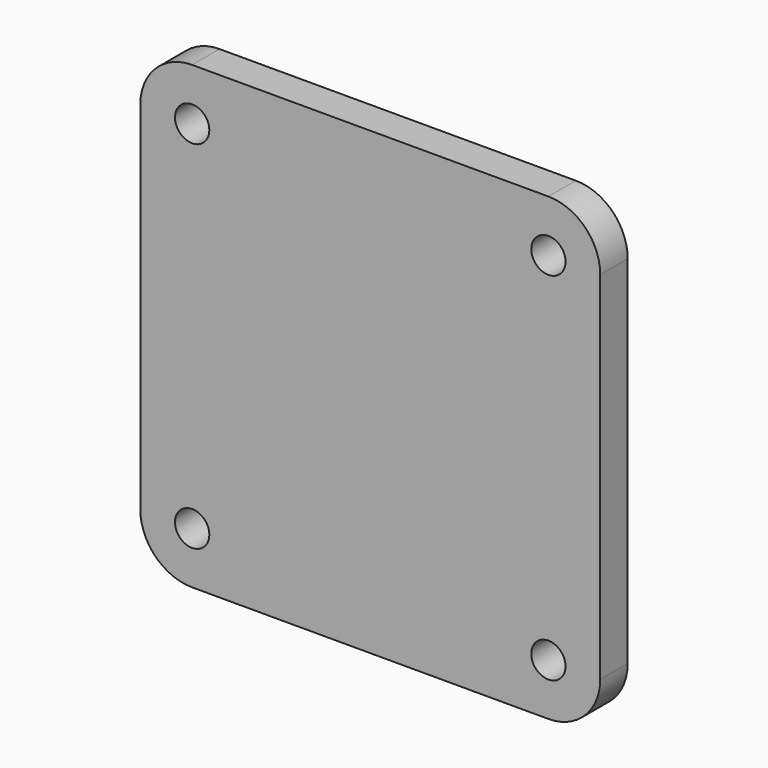
from build123d import *

# Parameters (mm, degrees)
F0_R     = 9.525
F1_DEPTH = 19.05


# Not quite as in the source:
# - a feature names something its author has since deleted; it is built from what else it names


with BuildPart() as f1:
    # F0 (on Front) → F1 (new body)
    with BuildSketch(Plane.XZ):
        with BuildLine():
            ThreePointArc((0, 28.7803760395), (8.4295769769, 8.4295769769), (28.7803760395, 0))
            Line((28.7803760395, 0), (226.5193760395, 0))
            ThreePointArc((226.5193760395, 0), (246.8701751021, 8.4295769769), (255.299752079, 28.7803760395))
            Line((255.299752079, 28.7803760395), (255.299752079, 226.5193760395))
            ThreePointArc((255.299752079, 226.5193760395), (246.8701751021, 246.8701751021), (226.5193760395, 255.299752079))
            Line((226.5193760395, 255.299752079), (28.7803760395, 255.299752079))
            ThreePointArc((28.7803760395, 255.299752079), (8.4295769769, 246.8701751021), (0, 226.5193760395))
            Line((0, 226.5193760395), (0, 28.7803760395))
        make_face()
        with Locations((28.7803760395, 28.7803760395)):
            Circle(F0_R, mode=Mode.SUBTRACT)
        with Locations((226.5193760395, 28.7803760395)):
            Circle(F0_R, mode=Mode.SUBTRACT)
        with Locations((28.7803760395, 226.5193760395)):
            Circle(F0_R, mode=Mode.SUBTRACT)
        with Locations((226.5193760395, 226.5193760395)):
            Circle(F0_R, mode=Mode.SUBTRACT)
    extrude(amount=F1_DEPTH)


solid = f1.part
